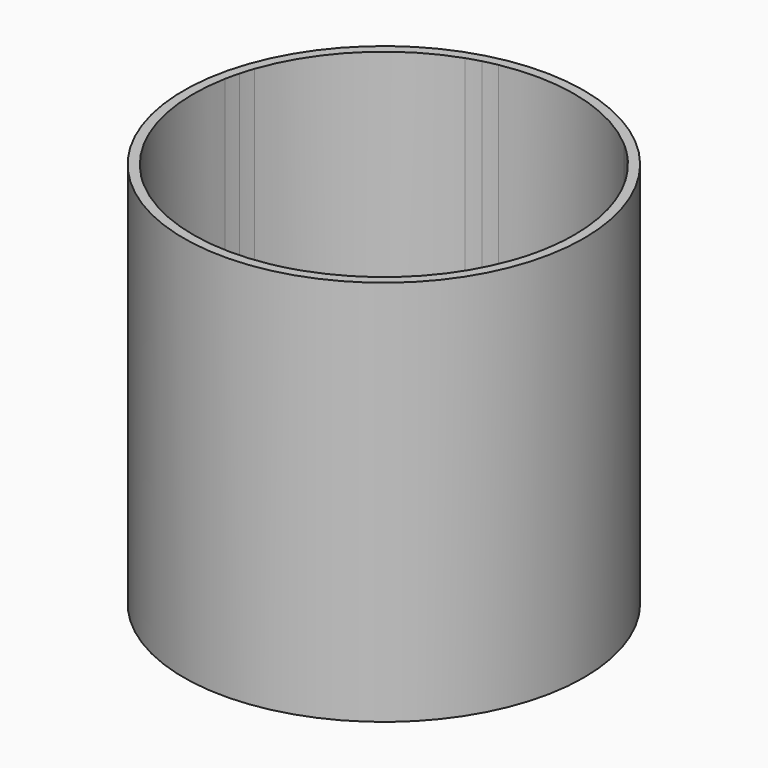
from build123d import *

# Parameters (mm, degrees)
F0_R     = 36.75
F1_DEPTH = 9
F2_DEPTH = 62
F3_DEPTH = 2.5
F4_DEPTH = 4


# Not quite as in the source:
# - a feature names something its author has since deleted; it is built from what else it names


with BuildPart() as f1:
    # F0 (on Top) → F1 (new body)
    with BuildSketch(Plane.XY):
        Circle(F0_R)
        with BuildLine():
            ThreePointArc((26.5730867913, 22.7787413695), (32.825737141, 12.1437630556), (35, 0))
            ThreePointArc((35, 0), (34.847012146, -3.2689057028), (34.3893860289, -6.5092340988))
            ThreePointArc((34.3893860289, -6.5092340988), (34.1183133858, -7.8064519285), (33.7983260972, -9.0924778266))
            ThreePointArc((33.7983260972, -9.0924778266), (33.4298829217, -10.3654680472), (33.0135120879, -11.6235975335))
            ThreePointArc((33.0135120879, -11.6235975335), (24.7239700923, -24.7734798298), (11.5575309257, -33.036698971))
            ThreePointArc((11.5575309257, -33.036698971), (10.2985710094, -33.4505520906), (9.0248462674, -33.8164479189))
            ThreePointArc((9.0248462674, -33.8164479189), (7.7381828098, -34.1338618794), (6.4404252966, -34.402338903))
            ThreePointArc((6.4404252966, -34.402338903), (-9.0924778266, -33.7983260972), (-22.8318551032, -26.5274648722))
            ThreePointArc((-22.8318551032, -26.5274648722), (-23.8197423763, -25.6441001621), (-24.7734798298, -24.7239700923))
            ThreePointArc((-24.7734798298, -24.7239700923), (-25.6917001119, -23.7683938321), (-26.5730867913, -22.7787413695))
            ThreePointArc((-26.5730867913, -22.7787413695), (-33.8164479189, -9.0248462674), (-34.3893860289, 6.5092340988))
            ThreePointArc((-34.3893860289, 6.5092340988), (-34.1183133858, 7.8064519285), (-33.7983260972, 9.0924778266))
            ThreePointArc((-33.7983260972, 9.0924778266), (-33.4298829217, 10.3654680472), (-33.0135120879, 11.6235975335))
            ThreePointArc((-33.0135120879, 11.6235975335), (-24.7239700923, 24.7734798298), (-11.5575309257, 33.036698971))
            ThreePointArc((-11.5575309257, 33.036698971), (-10.2985710094, 33.4505520906), (-9.0248462674, 33.8164479189))
            ThreePointArc((-9.0248462674, 33.8164479189), (-7.7381828098, 34.1338618794), (-6.4404252966, 34.402338903))
            ThreePointArc((-6.4404252966, 34.402338903), (9.0924778266, 33.7983260972), (22.8318551032, 26.5274648722))
            ThreePointArc((22.8318551032, 26.5274648722), (23.8197423763, 25.6441001621), (24.7734798298, 24.7239700923))
            ThreePointArc((24.7734798298, 24.7239700923), (25.6917001119, 23.7683938321), (26.5730867913, 22.7787413695))
        make_face(mode=Mode.SUBTRACT)
    extrude(amount=-F1_DEPTH)

    # F0 (on Top) → F2 (join)
    with BuildSketch(Plane.XY):
        Circle(F0_R)
        with BuildLine():
            ThreePointArc((26.5730867913, 22.7787413695), (32.825737141, 12.1437630556), (35, 0))
            ThreePointArc((35, 0), (34.847012146, -3.2689057028), (34.3893860289, -6.5092340988))
            ThreePointArc((34.3893860289, -6.5092340988), (34.1183133858, -7.8064519285), (33.7983260972, -9.0924778266))
            ThreePointArc((33.7983260972, -9.0924778266), (33.4298829217, -10.3654680472), (33.0135120879, -11.6235975335))
            ThreePointArc((33.0135120879, -11.6235975335), (24.7239700923, -24.7734798298), (11.5575309257, -33.036698971))
            ThreePointArc((11.5575309257, -33.036698971), (10.2985710094, -33.4505520906), (9.0248462674, -33.8164479189))
            ThreePointArc((9.0248462674, -33.8164479189), (7.7381828098, -34.1338618794), (6.4404252966, -34.402338903))
            ThreePointArc((6.4404252966, -34.402338903), (-9.0924778266, -33.7983260972), (-22.8318551032, -26.5274648722))
            ThreePointArc((-22.8318551032, -26.5274648722), (-23.8197423763, -25.6441001621), (-24.7734798298, -24.7239700923))
            ThreePointArc((-24.7734798298, -24.7239700923), (-25.6917001119, -23.7683938321), (-26.5730867913, -22.7787413695))
            ThreePointArc((-26.5730867913, -22.7787413695), (-33.8164479189, -9.0248462674), (-34.3893860289, 6.5092340988))
            ThreePointArc((-34.3893860289, 6.5092340988), (-34.1183133858, 7.8064519285), (-33.7983260972, 9.0924778266))
            ThreePointArc((-33.7983260972, 9.0924778266), (-33.4298829217, 10.3654680472), (-33.0135120879, 11.6235975335))
            ThreePointArc((-33.0135120879, 11.6235975335), (-24.7239700923, 24.7734798298), (-11.5575309257, 33.036698971))
            ThreePointArc((-11.5575309257, 33.036698971), (-10.2985710094, 33.4505520906), (-9.0248462674, 33.8164479189))
            ThreePointArc((-9.0248462674, 33.8164479189), (-7.7381828098, 34.1338618794), (-6.4404252966, 34.402338903))
            ThreePointArc((-6.4404252966, 34.402338903), (9.0924778266, 33.7983260972), (22.8318551032, 26.5274648722))
            ThreePointArc((22.8318551032, 26.5274648722), (23.8197423763, 25.6441001621), (24.7734798298, 24.7239700923))
            ThreePointArc((24.7734798298, 24.7239700923), (25.6917001119, 23.7683938321), (26.5730867913, 22.7787413695))
        make_face(mode=Mode.SUBTRACT)
    extrude(amount=F2_DEPTH)

    # F0 (on Top) → F3 (join)
    with BuildSketch(Plane.XY):
        with BuildLine():
            ThreePointArc((-10.9005525974, 31.9444901833), (-11.2956848318, 32.4505078709), (-11.5575309257, 33.036698971))
            ThreePointArc((-11.5575309257, 33.036698971), (-24.7239700923, 24.7734798298), (-33.0135120879, 11.6235975335))
            ThreePointArc((-33.0135120879, 11.6235975335), (-32.4278459824, 11.3605792915), (-31.9226197672, 10.9644355621))
            Line((-31.9226197672, 10.9644355621), (-28.1008002305, 14.7786172021))
            ThreePointArc((-28.1008002305, 14.7786172021), (-22.4281728694, 22.4730852741), (-14.7223721342, 28.1303085433))
            Line((-14.7223721342, 28.1303085433), (-10.9005525974, 31.9444901833))
        make_face()
        with BuildLine():
            ThreePointArc((-31.7227478819, 1.3152059995), (-30.6599101025, 8.2481763141), (-28.1008002305, 14.7786172021))
            Line((-28.1008002305, 14.7786172021), (-31.9226197672, 10.9644355621))
            ThreePointArc((-31.9226197672, 10.9644355621), (-31.2393099784, 8.4040473626), (-33.1150163084, 6.532089627))
            Line((-33.1150163084, 6.532089627), (-31.7227478819, 1.3152059995))
        make_face()
        with BuildLine():
            ThreePointArc((-26.8490580451, -16.9466982652), (-30.6763491835, -8.1868248283), (-31.7227478819, 1.3152059995))
            Line((-31.7227478819, 1.3152059995), (-33.1150163084, 6.532089627))
            ThreePointArc((-33.1150163084, 6.532089627), (-33.7508065978, 6.442903918), (-34.3893860289, 6.5092340988))
            ThreePointArc((-34.3893860289, 6.5092340988), (-33.8164479189, -9.0248462674), (-26.5730867913, -22.7787413695))
            ThreePointArc((-26.5730867913, -22.7787413695), (-26.0524732593, -22.4030487651), (-25.4567896186, -22.1635818927))
            Line((-25.4567896186, -22.1635818927), (-26.8490580451, -16.9466982652))
        make_face()
        with BuildLine():
            Line((-31.9226197672, 10.9644355621), (-33.7983260972, 9.0924778266))
            Line((-33.7983260972, 9.0924778266), (-33.1150163084, 6.532089627))
            ThreePointArc((-33.1150163084, 6.532089627), (-31.2393099784, 8.4040473626), (-31.9226197672, 10.9644355621))
        make_face()
        with BuildLine():
            ThreePointArc((-31.9226197672, 10.9644355621), (-32.4278459824, 11.3605792915), (-33.0135120879, 11.6235975335))
            ThreePointArc((-33.0135120879, 11.6235975335), (-33.4298829217, 10.3654680472), (-33.7983260972, 9.0924778266))
            Line((-33.7983260972, 9.0924778266), (-31.9226197672, 10.9644355621))
        make_face()
        with BuildLine():
            Line((-33.1150163084, 6.532089627), (-33.7983260972, 9.0924778266))
            ThreePointArc((-33.7983260972, 9.0924778266), (-34.1183133858, 7.8064519285), (-34.3893860289, 6.5092340988))
            ThreePointArc((-34.3893860289, 6.5092340988), (-33.7508065978, 6.442903918), (-33.1150163084, 6.532089627))
        make_face()
        with BuildLine():
            Line((-22.214463711, -25.4124005563), (-17.0003757477, -26.8151025438))
            ThreePointArc((-17.0003757477, -26.8151025438), (-22.4730852741, -22.4281728694), (-26.8490580451, -16.9466982652))
            Line((-26.8490580451, -16.9466982652), (-25.4567896186, -22.1635818927))
            ThreePointArc((-25.4567896186, -22.1635818927), (-22.8977734998, -22.8520123567), (-22.214463711, -25.4124005563))
        make_face()
        with BuildLine():
            ThreePointArc((-22.8318551032, -26.5274648722), (-9.0924778266, -33.7983260972), (6.4404252966, -34.402338903))
            ThreePointArc((6.4404252966, -34.402338903), (6.3753727231, -33.7636280565), (6.4658301487, -33.1280174548))
            Line((6.4658301487, -33.1280174548), (1.2517421854, -31.7253154673))
            ThreePointArc((1.2517421854, -31.7253154673), (-8.2481763141, -30.6599101025), (-17.0003757477, -26.8151025438))
            Line((-17.0003757477, -26.8151025438), (-22.214463711, -25.4124005563))
            ThreePointArc((-22.214463711, -25.4124005563), (-22.455121766, -26.0076039529), (-22.8318551032, -26.5274648722))
        make_face()
        with BuildLine():
            Line((-25.4567896186, -22.1635818927), (-24.7734798298, -24.7239700923))
            Line((-24.7734798298, -24.7239700923), (-22.214463711, -25.4124005563))
            ThreePointArc((-22.214463711, -25.4124005563), (-22.8977734998, -22.8520123567), (-25.4567896186, -22.1635818927))
        make_face()
        with BuildLine():
            ThreePointArc((-24.7734798298, -24.7239700923), (-23.8197423763, -25.6441001621), (-22.8318551032, -26.5274648722))
            ThreePointArc((-22.8318551032, -26.5274648722), (-22.455121766, -26.0076039529), (-22.214463711, -25.4124005563))
            Line((-22.214463711, -25.4124005563), (-24.7734798298, -24.7239700923))
        make_face()
        with BuildLine():
            ThreePointArc((-26.5730867913, -22.7787413695), (-25.6917001119, -23.7683938321), (-24.7734798298, -24.7239700923))
            Line((-24.7734798298, -24.7239700923), (-25.4567896186, -22.1635818927))
            ThreePointArc((-25.4567896186, -22.1635818927), (-26.0524732593, -22.4030487651), (-26.5730867913, -22.7787413695))
        make_face()
        with BuildLine():
            ThreePointArc((6.4658301487, -33.1280174548), (8.3415364786, -31.2560597193), (10.9005525974, -31.9444901833))
            Line((10.9005525974, -31.9444901833), (14.7223721342, -28.1303085433))
            ThreePointArc((14.7223721342, -28.1303085433), (8.1868248283, -30.6763491835), (1.2517421854, -31.7253154673))
            Line((1.2517421854, -31.7253154673), (6.4658301487, -33.1280174548))
        make_face()
        with BuildLine():
            ThreePointArc((6.4404252966, -34.402338903), (7.7381828098, -34.1338618794), (9.0248462674, -33.8164479189))
            Line((9.0248462674, -33.8164479189), (6.4658301487, -33.1280174548))
            ThreePointArc((6.4658301487, -33.1280174548), (6.3753727231, -33.7636280565), (6.4404252966, -34.402338903))
        make_face()
        with BuildLine():
            Line((6.4658301487, -33.1280174548), (9.0248462674, -33.8164479189))
            Line((9.0248462674, -33.8164479189), (10.9005525974, -31.9444901833))
            ThreePointArc((10.9005525974, -31.9444901833), (8.3415364786, -31.2560597193), (6.4658301487, -33.1280174548))
        make_face()
        with BuildLine():
            ThreePointArc((9.0248462674, -33.8164479189), (10.2985710094, -33.4505520906), (11.5575309257, -33.036698971))
            ThreePointArc((11.5575309257, -33.036698971), (11.2956848318, -32.4505078709), (10.9005525974, -31.9444901833))
            Line((10.9005525974, -31.9444901833), (9.0248462674, -33.8164479189))
        make_face()
        with BuildLine():
            ThreePointArc((11.5575309257, -33.036698971), (24.7239700923, -24.7734798298), (33.0135120879, -11.6235975335))
            ThreePointArc((33.0135120879, -11.6235975335), (32.4278459824, -11.3605792915), (31.9226197672, -10.9644355621))
            Line((31.9226197672, -10.9644355621), (28.1008002305, -14.7786172021))
            ThreePointArc((28.1008002305, -14.7786172021), (22.4281728694, -22.4730852741), (14.7223721342, -28.1303085433))
            Line((14.7223721342, -28.1303085433), (10.9005525974, -31.9444901833))
            ThreePointArc((10.9005525974, -31.9444901833), (11.2956848318, -32.4505078709), (11.5575309257, -33.036698971))
        make_face()
        with BuildLine():
            ThreePointArc((31.9226197672, -10.9644355621), (31.2393099784, -8.4040473626), (33.1150163084, -6.532089627))
            Line((33.1150163084, -6.532089627), (31.7227478819, -1.3152059995))
            ThreePointArc((31.7227478819, -1.3152059995), (30.6599101025, -8.2481763141), (28.1008002305, -14.7786172021))
            Line((28.1008002305, -14.7786172021), (31.9226197672, -10.9644355621))
        make_face()
        with BuildLine():
            Line((31.9226197672, -10.9644355621), (33.7983260972, -9.0924778266))
            Line((33.7983260972, -9.0924778266), (33.1150163084, -6.532089627))
            ThreePointArc((33.1150163084, -6.532089627), (31.2393099784, -8.4040473626), (31.9226197672, -10.9644355621))
        make_face()
        with BuildLine():
            ThreePointArc((33.0135120879, -11.6235975335), (33.4298829217, -10.3654680472), (33.7983260972, -9.0924778266))
            Line((33.7983260972, -9.0924778266), (31.9226197672, -10.9644355621))
            ThreePointArc((31.9226197672, -10.9644355621), (32.4278459824, -11.3605792915), (33.0135120879, -11.6235975335))
        make_face()
        with BuildLine():
            ThreePointArc((33.7983260972, -9.0924778266), (34.1183133858, -7.8064519285), (34.3893860289, -6.5092340988))
            ThreePointArc((34.3893860289, -6.5092340988), (33.7508065978, -6.442903918), (33.1150163084, -6.532089627))
            Line((33.1150163084, -6.532089627), (33.7983260972, -9.0924778266))
        make_face()
        with BuildLine():
            ThreePointArc((34.3893860289, -6.5092340988), (34.847012146, -3.2689057028), (35, 0))
            ThreePointArc((35, 0), (32.825737141, 12.1437630556), (26.5730867913, 22.7787413695))
            ThreePointArc((26.5730867913, 22.7787413695), (26.0524732593, 22.4030487651), (25.4567896186, 22.1635818927))
            Line((25.4567896186, 22.1635818927), (26.8490580451, 16.9466982652))
            ThreePointArc((26.8490580451, 16.9466982652), (30.5001646957, 8.8205699098), (31.75, 0))
            ThreePointArc((31.75, 0), (31.7431862393, -0.657744156), (31.7227478819, -1.3152059995))
            Line((31.7227478819, -1.3152059995), (33.1150163084, -6.532089627))
            ThreePointArc((33.1150163084, -6.532089627), (33.7508065978, -6.442903918), (34.3893860289, -6.5092340988))
        make_face()
        with BuildLine():
            Line((26.8490580451, 16.9466982652), (25.4567896186, 22.1635818927))
            ThreePointArc((25.4567896186, 22.1635818927), (22.8977734998, 22.8520123567), (22.214463711, 25.4124005563))
            Line((22.214463711, 25.4124005563), (17.0003757477, 26.8151025438))
            ThreePointArc((17.0003757477, 26.8151025438), (22.4730852741, 22.4281728694), (26.8490580451, 16.9466982652))
        make_face()
        with BuildLine():
            Line((25.4567896186, 22.1635818927), (24.7734798298, 24.7239700923))
            Line((24.7734798298, 24.7239700923), (22.214463711, 25.4124005563))
            ThreePointArc((22.214463711, 25.4124005563), (22.8977734998, 22.8520123567), (25.4567896186, 22.1635818927))
        make_face()
        with BuildLine():
            ThreePointArc((25.4567896186, 22.1635818927), (26.0524732593, 22.4030487651), (26.5730867913, 22.7787413695))
            ThreePointArc((26.5730867913, 22.7787413695), (25.6917001119, 23.7683938321), (24.7734798298, 24.7239700923))
            Line((24.7734798298, 24.7239700923), (25.4567896186, 22.1635818927))
        make_face()
        with BuildLine():
            Line((22.214463711, 25.4124005563), (24.7734798298, 24.7239700923))
            ThreePointArc((24.7734798298, 24.7239700923), (23.8197423763, 25.6441001621), (22.8318551032, 26.5274648722))
            ThreePointArc((22.8318551032, 26.5274648722), (22.455121766, 26.0076039529), (22.214463711, 25.4124005563))
        make_face()
        with BuildLine():
            ThreePointArc((22.214463711, 25.4124005563), (22.455121766, 26.0076039529), (22.8318551032, 26.5274648722))
            ThreePointArc((22.8318551032, 26.5274648722), (9.0924778266, 33.7983260972), (-6.4404252966, 34.402338903))
            ThreePointArc((-6.4404252966, 34.402338903), (-6.3753727231, 33.7636280565), (-6.4658301487, 33.1280174548))
            Line((-6.4658301487, 33.1280174548), (-1.2517421854, 31.7253154673))
            ThreePointArc((-1.2517421854, 31.7253154673), (8.2481763141, 30.6599101025), (17.0003757477, 26.8151025438))
            Line((17.0003757477, 26.8151025438), (22.214463711, 25.4124005563))
        make_face()
        with BuildLine():
            Line((-1.2517421854, 31.7253154673), (-6.4658301487, 33.1280174548))
            ThreePointArc((-6.4658301487, 33.1280174548), (-8.3415364786, 31.2560597193), (-10.9005525974, 31.9444901833))
            Line((-10.9005525974, 31.9444901833), (-14.7223721342, 28.1303085433))
            ThreePointArc((-14.7223721342, 28.1303085433), (-8.1868248283, 30.6763491835), (-1.2517421854, 31.7253154673))
        make_face()
        with BuildLine():
            Line((-6.4658301487, 33.1280174548), (-9.0248462674, 33.8164479189))
            Line((-9.0248462674, 33.8164479189), (-10.9005525974, 31.9444901833))
            ThreePointArc((-10.9005525974, 31.9444901833), (-8.3415364786, 31.2560597193), (-6.4658301487, 33.1280174548))
        make_face()
        with BuildLine():
            Line((-10.9005525974, 31.9444901833), (-9.0248462674, 33.8164479189))
            ThreePointArc((-9.0248462674, 33.8164479189), (-10.2985710094, 33.4505520906), (-11.5575309257, 33.036698971))
            ThreePointArc((-11.5575309257, 33.036698971), (-11.2956848318, 32.4505078709), (-10.9005525974, 31.9444901833))
        make_face()
        with BuildLine():
            ThreePointArc((-6.4658301487, 33.1280174548), (-6.3753727231, 33.7636280565), (-6.4404252966, 34.402338903))
            ThreePointArc((-6.4404252966, 34.402338903), (-7.7381828098, 34.1338618794), (-9.0248462674, 33.8164479189))
            Line((-9.0248462674, 33.8164479189), (-6.4658301487, 33.1280174548))
        make_face()
    extrude(amount=F3_DEPTH)

    # F0 (on Top) → F4 (join)
    with BuildSketch(Plane.XY):
        with BuildLine():
            Line((6.4658301487, -33.1280174548), (9.0248462674, -33.8164479189))
            Line((9.0248462674, -33.8164479189), (10.9005525974, -31.9444901833))
            ThreePointArc((10.9005525974, -31.9444901833), (8.3415364786, -31.2560597193), (6.4658301487, -33.1280174548))
        make_face()
        with BuildLine():
            ThreePointArc((9.0248462674, -33.8164479189), (10.2985710094, -33.4505520906), (11.5575309257, -33.036698971))
            ThreePointArc((11.5575309257, -33.036698971), (11.2956848318, -32.4505078709), (10.9005525974, -31.9444901833))
            Line((10.9005525974, -31.9444901833), (9.0248462674, -33.8164479189))
        make_face()
        with BuildLine():
            ThreePointArc((6.4404252966, -34.402338903), (7.7381828098, -34.1338618794), (9.0248462674, -33.8164479189))
            Line((9.0248462674, -33.8164479189), (6.4658301487, -33.1280174548))
            ThreePointArc((6.4658301487, -33.1280174548), (6.3753727231, -33.7636280565), (6.4404252966, -34.402338903))
        make_face()
        with BuildLine():
            ThreePointArc((-26.5730867913, -22.7787413695), (-25.6917001119, -23.7683938321), (-24.7734798298, -24.7239700923))
            Line((-24.7734798298, -24.7239700923), (-25.4567896186, -22.1635818927))
            ThreePointArc((-25.4567896186, -22.1635818927), (-26.0524732593, -22.4030487651), (-26.5730867913, -22.7787413695))
        make_face()
        with BuildLine():
            Line((-25.4567896186, -22.1635818927), (-24.7734798298, -24.7239700923))
            Line((-24.7734798298, -24.7239700923), (-22.214463711, -25.4124005563))
            ThreePointArc((-22.214463711, -25.4124005563), (-22.8977734998, -22.8520123567), (-25.4567896186, -22.1635818927))
        make_face()
        with BuildLine():
            ThreePointArc((-24.7734798298, -24.7239700923), (-23.8197423763, -25.6441001621), (-22.8318551032, -26.5274648722))
            ThreePointArc((-22.8318551032, -26.5274648722), (-22.455121766, -26.0076039529), (-22.214463711, -25.4124005563))
            Line((-22.214463711, -25.4124005563), (-24.7734798298, -24.7239700923))
        make_face()
        with BuildLine():
            ThreePointArc((-31.9226197672, 10.9644355621), (-32.4278459824, 11.3605792915), (-33.0135120879, 11.6235975335))
            ThreePointArc((-33.0135120879, 11.6235975335), (-33.4298829217, 10.3654680472), (-33.7983260972, 9.0924778266))
            Line((-33.7983260972, 9.0924778266), (-31.9226197672, 10.9644355621))
        make_face()
        with BuildLine():
            Line((-31.9226197672, 10.9644355621), (-33.7983260972, 9.0924778266))
            Line((-33.7983260972, 9.0924778266), (-33.1150163084, 6.532089627))
            ThreePointArc((-33.1150163084, 6.532089627), (-31.2393099784, 8.4040473626), (-31.9226197672, 10.9644355621))
        make_face()
        with BuildLine():
            Line((-33.1150163084, 6.532089627), (-33.7983260972, 9.0924778266))
            ThreePointArc((-33.7983260972, 9.0924778266), (-34.1183133858, 7.8064519285), (-34.3893860289, 6.5092340988))
            ThreePointArc((-34.3893860289, 6.5092340988), (-33.7508065978, 6.442903918), (-33.1150163084, 6.532089627))
        make_face()
        with BuildLine():
            Line((-6.4658301487, 33.1280174548), (-9.0248462674, 33.8164479189))
            Line((-9.0248462674, 33.8164479189), (-10.9005525974, 31.9444901833))
            ThreePointArc((-10.9005525974, 31.9444901833), (-8.3415364786, 31.2560597193), (-6.4658301487, 33.1280174548))
        make_face()
        with BuildLine():
            ThreePointArc((-6.4658301487, 33.1280174548), (-6.3753727231, 33.7636280565), (-6.4404252966, 34.402338903))
            ThreePointArc((-6.4404252966, 34.402338903), (-7.7381828098, 34.1338618794), (-9.0248462674, 33.8164479189))
            Line((-9.0248462674, 33.8164479189), (-6.4658301487, 33.1280174548))
        make_face()
        with BuildLine():
            Line((-10.9005525974, 31.9444901833), (-9.0248462674, 33.8164479189))
            ThreePointArc((-9.0248462674, 33.8164479189), (-10.2985710094, 33.4505520906), (-11.5575309257, 33.036698971))
            ThreePointArc((-11.5575309257, 33.036698971), (-11.2956848318, 32.4505078709), (-10.9005525974, 31.9444901833))
        make_face()
        with BuildLine():
            Line((22.214463711, 25.4124005563), (24.7734798298, 24.7239700923))
            ThreePointArc((24.7734798298, 24.7239700923), (23.8197423763, 25.6441001621), (22.8318551032, 26.5274648722))
            ThreePointArc((22.8318551032, 26.5274648722), (22.455121766, 26.0076039529), (22.214463711, 25.4124005563))
        make_face()
        with BuildLine():
            Line((25.4567896186, 22.1635818927), (24.7734798298, 24.7239700923))
            Line((24.7734798298, 24.7239700923), (22.214463711, 25.4124005563))
            ThreePointArc((22.214463711, 25.4124005563), (22.8977734998, 22.8520123567), (25.4567896186, 22.1635818927))
        make_face()
        with BuildLine():
            ThreePointArc((25.4567896186, 22.1635818927), (26.0524732593, 22.4030487651), (26.5730867913, 22.7787413695))
            ThreePointArc((26.5730867913, 22.7787413695), (25.6917001119, 23.7683938321), (24.7734798298, 24.7239700923))
            Line((24.7734798298, 24.7239700923), (25.4567896186, 22.1635818927))
        make_face()
        with BuildLine():
            Line((31.9226197672, -10.9644355621), (33.7983260972, -9.0924778266))
            Line((33.7983260972, -9.0924778266), (33.1150163084, -6.532089627))
            ThreePointArc((33.1150163084, -6.532089627), (31.2393099784, -8.4040473626), (31.9226197672, -10.9644355621))
        make_face()
        with BuildLine():
            ThreePointArc((33.7983260972, -9.0924778266), (34.1183133858, -7.8064519285), (34.3893860289, -6.5092340988))
            ThreePointArc((34.3893860289, -6.5092340988), (33.7508065978, -6.442903918), (33.1150163084, -6.532089627))
            Line((33.1150163084, -6.532089627), (33.7983260972, -9.0924778266))
        make_face()
        with BuildLine():
            ThreePointArc((33.0135120879, -11.6235975335), (33.4298829217, -10.3654680472), (33.7983260972, -9.0924778266))
            Line((33.7983260972, -9.0924778266), (31.9226197672, -10.9644355621))
            ThreePointArc((31.9226197672, -10.9644355621), (32.4278459824, -11.3605792915), (33.0135120879, -11.6235975335))
        make_face()
    extrude(amount=F4_DEPTH)


solid = f1.part
